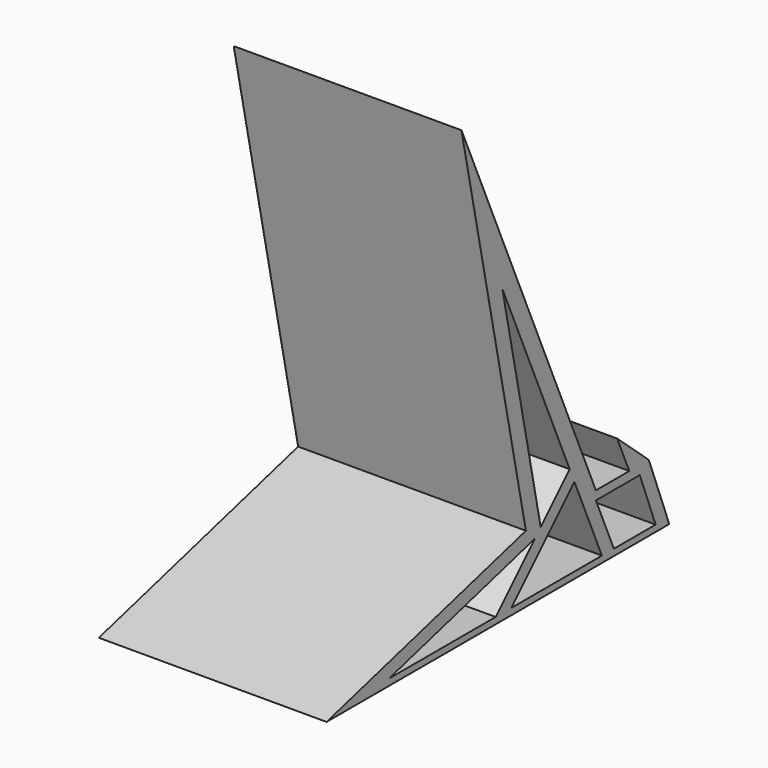
from build123d import *

# Parameters (mm, degrees)
F1_DEPTH = 60


# Not quite as in the source:
# - a feature names something its author has since deleted; it is built from what else it names


with BuildPart() as f1:
    # F0 (on Right) → F1 (new body)
    with BuildSketch(Plane.YZ):
        Polygon((-9.6511039816, 84.8569979519), (11.5631884334, -16.6570162717), (-54.0677122772, -34.3161821365), (58.7390847504, -34.3161821365), (57.1931600571, -30.1430020481), (52.030442059, -16.6570162717), (41.619012037, -7.4873352069), (45.6172674894, -16.6570162717), (45.6120451947, -16.6570162717), (34.6120451947, -16.6570162717), align=None)
        Polygon((-33.4832413232, -32.6066525748), (14.5474322128, -19.683142134), (1.6078982385, -32.6066525748), align=None, mode=Mode.SUBTRACT)
        Polygon((6.7093357808, -32.6066525748), (27.5331988357, -11.8085765279), (36.6017826139, -32.6066525748), align=None, mode=Mode.SUBTRACT)
        Polygon((34.5994135062, -18.9948312665), (45.6120451947, -18.9948312665), (49.0652749053, -18.9948312665), (54.2761653822, -32.6066525748), (40.534575087, -32.6066525748), (38.136206347, -27.1061845124), align=None, mode=Mode.SUBTRACT)
        Polygon((16.4317106992, -17.8011970237), (3.8088566841, 42.6013163841), (25.9855565835, -8.2591820422), align=None, mode=Mode.SUBTRACT)
    extrude(amount=F1_DEPTH)


solid = f1.part
